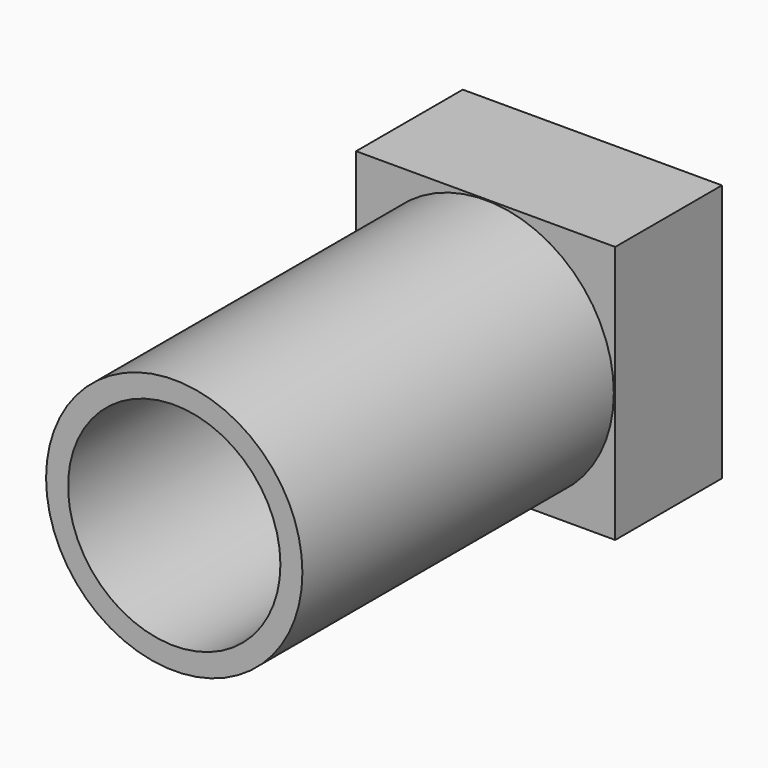
from build123d import *

# Parameters (mm, degrees)
F0_W     = 98.7017413428
F0_H     = 98.2726
F0_R     = 40.4346760416
F1_DEPTH = 50.8
F2_R     = 48.8166771829
F2_R_2   = 40.4346760416
F3_DEPTH = 148.2671336


# Not quite as in the source:
# - an extrude ends at something that could not be found from the text; its depth is read off the source's solid


with BuildPart() as f1:
    # F0 (on Front) → F1 (new body)
    with BuildSketch(Plane.XZ):
        Rectangle(F0_W, F0_H)
        Circle(F0_R, mode=Mode.SUBTRACT)
    extrude(amount=-F1_DEPTH)

    # F2 (on face) → F3 (join, through all)
    with BuildSketch(Plane.XZ):
        Circle(F2_R)
        Circle(F2_R_2, mode=Mode.SUBTRACT)
    extrude(amount=F3_DEPTH)


solid = f1.part
